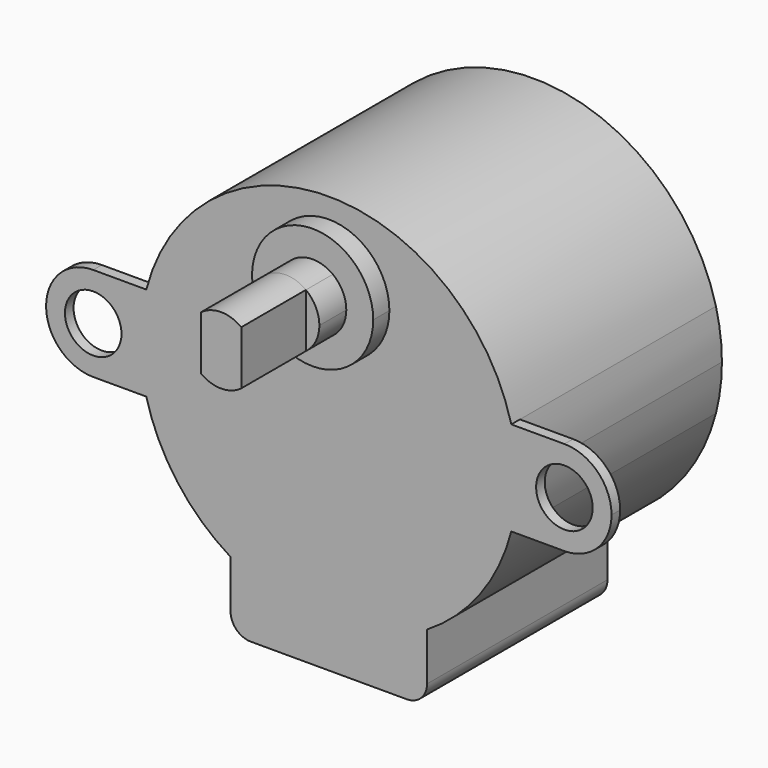
from build123d import *
from build123d import SkipClean  # not in build123d's __all__

# Parameters (mm, degrees)
F1_DEPTH = 1.5
F2_DEPTH = 19
F0_R     = 2.1
F3_DEPTH = 0.8
F4_DEPTH = 4
F5_DEPTH = 10
F6_DEPTH = 16.75
F7_R     = 1.5


with BuildPart() as f1:
    # F0 (on Front) → F1 (new body)
    with BuildSketch(Plane.XZ):
        with BuildLine():
            ThreePointArc((4.5, 8), (-3.1819805153, 11.1819805153), (0, 3.5))
            ThreePointArc((0, 3.5), (3.1819805153, 4.8180194847), (4.5, 8))
        make_face()
        with BuildLine():
            ThreePointArc((1.5, 6), (0.790569415, 5.6282917549), (0, 5.5))
            ThreePointArc((0, 5.5), (-0.790569415, 5.6282917549), (-1.5, 6))
            ThreePointArc((-1.5, 6), (-2.5, 8), (-1.5, 10))
            ThreePointArc((-1.5, 10), (0, 10.5), (1.5, 10))
            ThreePointArc((1.5, 10), (2.2360679775, 9.1180339887), (2.5, 8))
            ThreePointArc((2.5, 8), (2.2360679775, 6.8819660113), (1.5, 6))
        make_face(mode=Mode.SUBTRACT)
    extrude(amount=F1_DEPTH)

    # F0 (on Front) → F2 (join)
    with BuildSketch(Plane.XZ):
        with BuildLine():
            Line((0, 3.5), (13.5554417117, 3.5))
            ThreePointArc((13.5554417117, 3.5), (0, 14), (-13.5554417117, 3.5))
            Line((-13.5554417117, 3.5), (0, 3.5))
        make_face()
        with BuildLine():
            ThreePointArc((4.5, 8), (3.1819805153, 4.8180194847), (0, 3.5))
            ThreePointArc((0, 3.5), (-3.1819805153, 11.1819805153), (4.5, 8))
        make_face(mode=Mode.SUBTRACT)
        with BuildLine():
            ThreePointArc((-13.5554417117, -3.5), (-11.250406053, -8.3323684294), (-7.3, -11.9461290802))
            Line((-7.3, -11.9461290802), (-7.3, -3.5))
            Line((-7.3, -3.5), (-13.5554417117, -3.5))
        make_face()
        with BuildLine():
            ThreePointArc((4.5, 8), (-3.1819805153, 11.1819805153), (0, 3.5))
            ThreePointArc((0, 3.5), (3.1819805153, 4.8180194847), (4.5, 8))
        make_face()
        with BuildLine():
            ThreePointArc((1.5, 6), (0.790569415, 5.6282917549), (0, 5.5))
            ThreePointArc((0, 5.5), (-0.790569415, 5.6282917549), (-1.5, 6))
            ThreePointArc((-1.5, 6), (-2.5, 8), (-1.5, 10))
            ThreePointArc((-1.5, 10), (0, 10.5), (1.5, 10))
            ThreePointArc((1.5, 10), (2.2360679775, 9.1180339887), (2.5, 8))
            ThreePointArc((2.5, 8), (2.2360679775, 6.8819660113), (1.5, 6))
        make_face(mode=Mode.SUBTRACT)
        with BuildLine():
            ThreePointArc((-1.5, 10), (-2.5, 8), (-1.5, 6))
            Line((-1.5, 6), (-1.5, 10))
        make_face()
        with BuildLine():
            Line((1.5, 10), (1.5, 6))
            ThreePointArc((1.5, 6), (2.2360679775, 6.8819660113), (2.5, 8))
            ThreePointArc((2.5, 8), (2.2360679775, 9.1180339887), (1.5, 10))
        make_face()
        with BuildLine():
            ThreePointArc((-1.5, 6), (-0.790569415, 5.6282917549), (0, 5.5))
            ThreePointArc((0, 5.5), (0.790569415, 5.6282917549), (1.5, 6))
            Line((1.5, 6), (1.5, 10))
            ThreePointArc((1.5, 10), (0, 10.5), (-1.5, 10))
            Line((-1.5, 10), (-1.5, 6))
        make_face()
        with BuildLine():
            ThreePointArc((13.5554417117, -3.5), (13.8884157477, -1.7640600948), (14, 0))
            ThreePointArc((14, 0), (13.8884157477, 1.7640600948), (13.5554417117, 3.5))
            Line((13.5554417117, 3.5), (0, 3.5))
            Line((0, 3.5), (-13.5554417117, 3.5))
            ThreePointArc((-13.5554417117, 3.5), (-13.8884157477, 1.7640600948), (-14, 0))
            ThreePointArc((-14, 0), (-13.8884157477, -1.7640600948), (-13.5554417117, -3.5))
            Line((-13.5554417117, -3.5), (-7.3, -3.5))
            Line((-7.3, -3.5), (7.3, -3.5))
            Line((7.3, -3.5), (13.5554417117, -3.5))
        make_face()
        with BuildLine():
            ThreePointArc((-7.3, -11.9461290802), (0, -14), (7.3, -11.9461290802))
            Line((7.3, -11.9461290802), (7.3, -3.5))
            Line((7.3, -3.5), (-7.3, -3.5))
            Line((-7.3, -3.5), (-7.3, -11.9461290802))
        make_face()
        with BuildLine():
            ThreePointArc((7.3, -11.9461290802), (11.250406053, -8.3323684294), (13.5554417117, -3.5))
            Line((13.5554417117, -3.5), (7.3, -3.5))
            Line((7.3, -3.5), (7.3, -11.9461290802))
        make_face()
    extrude(amount=-F2_DEPTH)

    # F0 (on Front) → F3 (join)
    with BuildSketch(Plane.XZ):
        with BuildLine():
            ThreePointArc((-17.5, -3.5), (-15.0251262658, -2.4748737342), (-14, 0))
            ThreePointArc((-14, 0), (-15.0251262658, 2.4748737342), (-17.5, 3.5))
            ThreePointArc((-17.5, 3.5), (-21, 0), (-17.5, -3.5))
        make_face()
        with Locations((-17.5, 0)):
            Circle(F0_R, mode=Mode.SUBTRACT)
        with BuildLine():
            ThreePointArc((-14, 0), (-13.8884157477, 1.7640600948), (-13.5554417117, 3.5))
            Line((-13.5554417117, 3.5), (-17.5, 3.5))
            ThreePointArc((-17.5, 3.5), (-15.0251262658, 2.4748737342), (-14, 0))
        make_face()
        with BuildLine():
            ThreePointArc((-13.5554417117, -3.5), (-13.8884157477, -1.7640600948), (-14, 0))
            ThreePointArc((-14, 0), (-15.0251262658, -2.4748737342), (-17.5, -3.5))
            Line((-17.5, -3.5), (-13.5554417117, -3.5))
        make_face()
        with BuildLine():
            ThreePointArc((13.5554417117, 3.5), (13.8884157477, 1.7640600948), (14, 0))
            ThreePointArc((14, 0), (15.0251262658, 2.4748737342), (17.5, 3.5))
            Line((17.5, 3.5), (13.5554417117, 3.5))
        make_face()
        with BuildLine():
            ThreePointArc((17.5, 3.5), (15.0251262658, 2.4748737342), (14, 0))
            ThreePointArc((14, 0), (15.0251262658, -2.4748737342), (17.5, -3.5))
            ThreePointArc((17.5, -3.5), (19.9748737342, -2.4748737342), (21, 0))
            ThreePointArc((21, 0), (19.9748737342, 2.4748737342), (17.5, 3.5))
        make_face()
        with Locations((17.5, 0)):
            Circle(F0_R, mode=Mode.SUBTRACT)
        with BuildLine():
            ThreePointArc((17.5, -3.5), (15.0251262658, -2.4748737342), (14, 0))
            ThreePointArc((14, 0), (13.8884157477, -1.7640600948), (13.5554417117, -3.5))
            Line((13.5554417117, -3.5), (17.5, -3.5))
        make_face()
    extrude(amount=-F3_DEPTH)

    # F0 (on Front) → F6 (join)
    with BuildSketch(Plane.XZ):
        with BuildLine():
            Line((7.3, -17), (7.3, -11.9461290802))
            ThreePointArc((7.3, -11.9461290802), (0, -14), (-7.3, -11.9461290802))
            Line((-7.3, -11.9461290802), (-7.3, -17))
            Line((-7.3, -17), (7.3, -17))
        make_face()
    extrude(amount=-F6_DEPTH)

    # F7
    f7_edges = [f1.edges().sort_by_distance(p)[0] for p in [
        (-7.3, 8.375, -17),
        (7.3, 8.375, -17),
    ]]
    fillet(f7_edges, radius=F7_R)


with BuildPart() as f4:
    # F0 (on Front) → F4 (new body)
    with BuildSketch(Plane.XZ):
        with BuildLine():
            ThreePointArc((-1.5, 10), (-2.5, 8), (-1.5, 6))
            Line((-1.5, 6), (-1.5, 10))
        make_face()
        with BuildLine():
            ThreePointArc((-1.5, 6), (-0.790569415, 5.6282917549), (0, 5.5))
            ThreePointArc((0, 5.5), (0.790569415, 5.6282917549), (1.5, 6))
            Line((1.5, 6), (1.5, 10))
            ThreePointArc((1.5, 10), (0, 10.5), (-1.5, 10))
            Line((-1.5, 10), (-1.5, 6))
        make_face()
        with BuildLine():
            Line((1.5, 10), (1.5, 6))
            ThreePointArc((1.5, 6), (2.2360679775, 6.8819660113), (2.5, 8))
            ThreePointArc((2.5, 8), (2.2360679775, 9.1180339887), (1.5, 10))
        make_face()
    extrude(amount=F4_DEPTH)

    # F0 (on Front) → F5 (join)
    with BuildSketch(Plane.XZ):
        with BuildLine():
            ThreePointArc((-1.5, 6), (-0.790569415, 5.6282917549), (0, 5.5))
            ThreePointArc((0, 5.5), (0.790569415, 5.6282917549), (1.5, 6))
            Line((1.5, 6), (1.5, 10))
            ThreePointArc((1.5, 10), (0, 10.5), (-1.5, 10))
            Line((-1.5, 10), (-1.5, 6))
        make_face()
    with SkipClean():  # cleaning this boolean's faces spoils the solid; the shape is the same uncleaned
        extrude(amount=F5_DEPTH)


solid = Compound([f1.part, f4.part])
